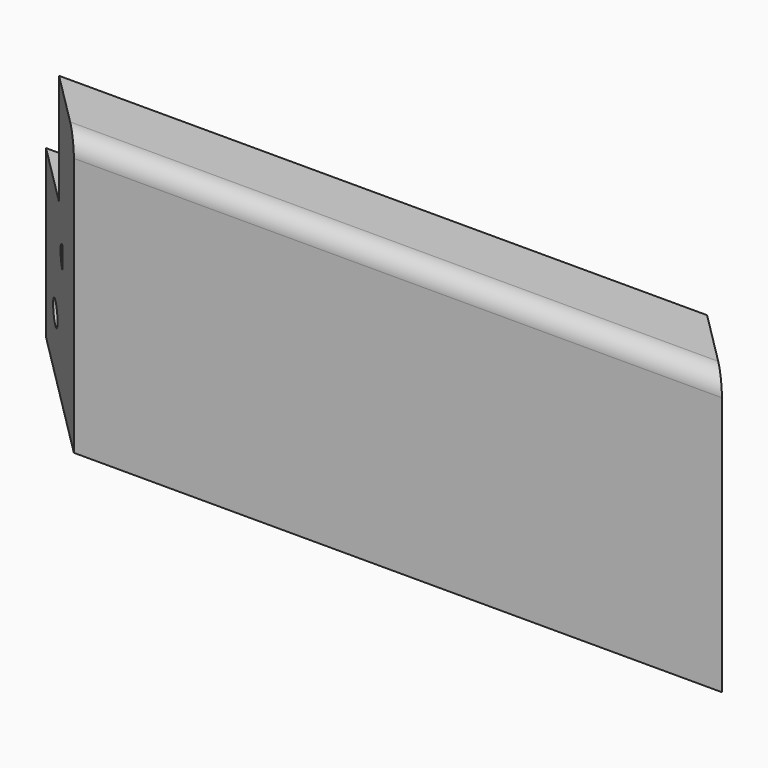
from build123d import *

# Parameters (mm, degrees)
F3_DEPTH = 215
F4_SIZE  = 79.99999
F5_R     = 6
F6_DEPTH = 50
F7_W     = 116
F7_H     = 90
F8_DEPTH = 5
F9_R     = 10


# Not quite as in the source:
# - a fillet or chamfer is up to 0.001 mm smaller than in the source, because OpenCascade refuses the exact size


with BuildPart() as f3:
    # F2 (on Right) → F3 (new body, symmetric)
    with BuildSketch(Plane.YZ):
        Polygon((-40, 75), (-40, -75), (40, -75), (40, 15), (0, 15), (0, 75), align=None)
    extrude(amount=F3_DEPTH, both=True)

    # F4 (size 80 in the source; OpenCascade refuses exactly that, so slightly less here)
    f4_edges = [f3.edges().sort_by_distance(p)[0] for p in [
        (215, 40, -30),
        (-215, -40, 0),
    ]]
    chamfer(f4_edges, length=F4_SIZE)

    # F5 (on face) → F6 (cut)
    with BuildSketch(Plane(origin=(0, 40, 0), x_dir=(-1, 0, 0), z_dir=(0, 1, 0))):
        with Locations((-105, -45)):
            Circle(F5_R)
        with Locations((-85, -5)):
            Circle(F5_R)
        with Locations((165, -5)):
            Circle(F5_R)
        with Locations((185, -45)):
            Circle(F5_R)
    extrude(amount=-F6_DEPTH, mode=Mode.SUBTRACT)

    # F7 (on face) → F8 (cut)
    with BuildSketch(Plane(origin=(0, 40, 0), x_dir=(-1, 0, 0), z_dir=(0, 1, 0))):
        with Locations((-117, -30)):
            Rectangle(F7_W, F7_H)
        with Locations((197, -30)):
            Rectangle(F7_W, F7_H)
    extrude(amount=-F8_DEPTH, mode=Mode.SUBTRACT)

    # F9
    f9_edges = [f3.edges().sort_by_distance(p)[0] for p in [
        (39.999995, -40, 75),
    ]]
    fillet(f9_edges, radius=F9_R)


solid = f3.part
